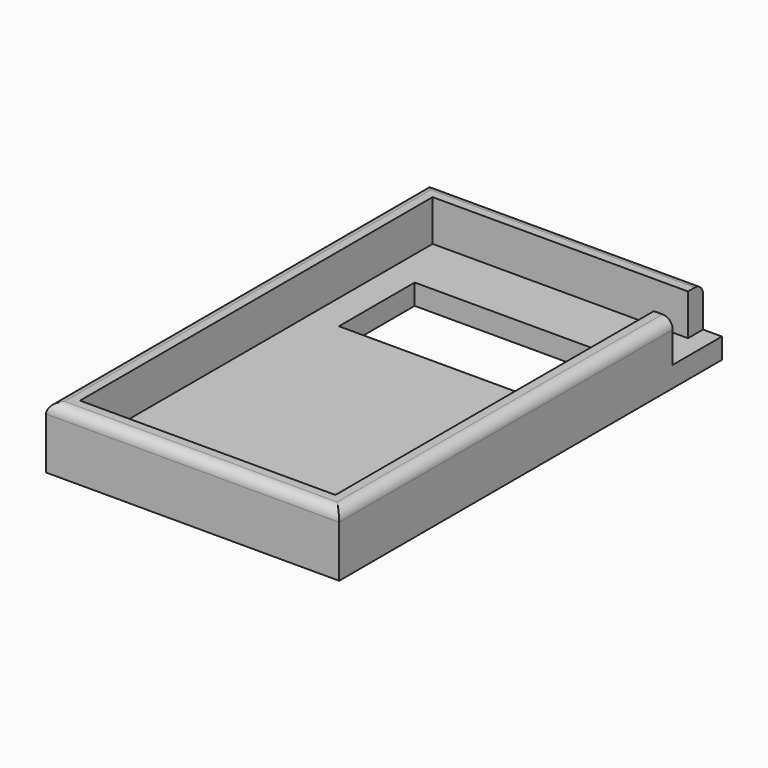
from build123d import *

# Parameters (mm, degrees)
F0_W     = 47.5
F0_H     = 23
F1_DEPTH = 5
F2_DEPTH = 15
F3_R     = 2.5


with BuildPart() as f1:
    # F0 (on Top) → F1 (new body)
    with BuildSketch(Plane.XY):
        Polygon((35.5799995661, 43.7052872479), (35.5799995661, 58.0799995661), (31, 58.0799995661), (31, 53.5), (31, 43.15), (35.5799995661, 43.15), align=None)
        Polygon((31, 53.5), (31, 58.0799995661), (-35.5799995661, 58.0799995661), (-35.5799995661, -58.0799995661), (35.5799995661, -58.0799995661), (35.5799995661, 43.15), (31, 43.15), (31, -53.5), (-31, -53.5), (-31, 53.5), align=None)
        Polygon((31, 43.15), (31, 53.5), (-31, 53.5), (-31, -53.5), (31, -53.5), align=None)
        with Locations((0, 27.5)):
            Rectangle(F0_W, F0_H, mode=Mode.SUBTRACT)
    extrude(amount=F1_DEPTH)

    # F0 (on Top) → F2 (join)
    with BuildSketch(Plane.XY):
        Polygon((31, 53.5), (31, 58.0799995661), (-35.5799995661, 58.0799995661), (-35.5799995661, -58.0799995661), (35.5799995661, -58.0799995661), (35.5799995661, 43.15), (31, 43.15), (31, -53.5), (-31, -53.5), (-31, 53.5), align=None)
    extrude(amount=F2_DEPTH)

    # F3
    f3_edges = [f1.edges().sort_by_distance(p)[0] for p in [
        (-35.58, 0, 15),
        (-2.29, 58.08, 15),
        (0, -58.08, 15),
        (35.58, -7.465, 15),
    ]]
    fillet(f3_edges, radius=F3_R)


solid = f1.part
